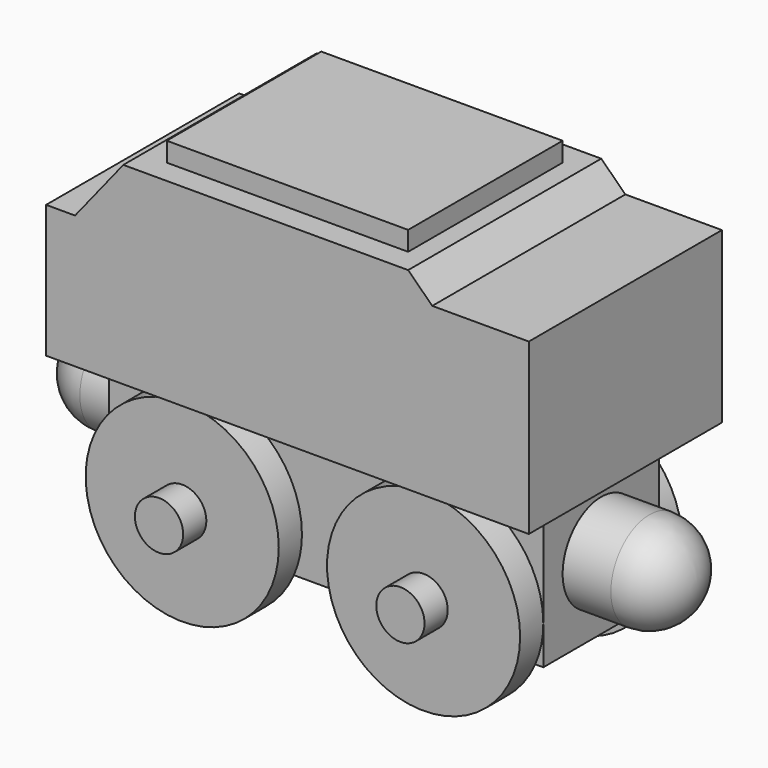
from build123d import *

# Parameters (mm, degrees)
F0_W      = 45
F0_H      = 15
F1_DEPTH  = 7.5
F2_W      = 50
F2_H      = 25
F3_DEPTH  = 20
F5_DEPTH  = 25
F7_DEPTH  = 25
F8_W      = 25
F8_H      = 20
F9_DEPTH  = 2
F11_W     = 5
F11_H     = 5
F13_W     = 5
F13_H     = 5
F15_R     = 10
F16_DEPTH = 3
F17_R     = 10
F18_DEPTH = 3
F19_R     = 2.5
F20_DEPTH = 3
F21_R     = 2.5
F22_DEPTH = 3


# Not quite as in the source:
# - a pattern or mirror of a feature is missing from the dataset's text; its kind, count and spacing are read off the source's solid


with BuildPart() as f1:
    # F0 (on Top) → F1 (new body, symmetric)
    with BuildSketch(Plane.XY):
        Rectangle(F0_W, F0_H)
    extrude(amount=F1_DEPTH, both=True)

    # F2 (on face) → F3 (join)
    with BuildSketch(Plane.XY.offset(7.5)):
        Rectangle(F2_W, F2_H)
    extrude(amount=F3_DEPTH)

    # F4 (on face) → F5 (cut, through all)
    with BuildSketch(Plane.XZ.offset(12.5)):
        Polygon((25, 27.5), (12.5, 27.5), (15, 25.0505102572), (25, 25.0505102572), align=None)
    extrude(amount=-F5_DEPTH, mode=Mode.SUBTRACT)

    # F6 (on face) → F7 (cut, through all)
    with BuildSketch(Plane.XZ.offset(12.5)):
        Polygon((-25, 27.5), (-25, 21.2550020016), (-22, 21.2550020016), (-17, 27.5), align=None)
    extrude(amount=-F7_DEPTH, mode=Mode.SUBTRACT)

    # F8 (on face) → F9 (join)
    with BuildSketch(Plane.XY.offset(27.5)):
        with Locations((-2, 0)):
            Rectangle(F8_W, F8_H)
    extrude(amount=F9_DEPTH)

    # F11 (on Front) → F12 (revolve)
    with BuildSketch(Plane.XZ):
        with Locations((25, -2.5)):
            Rectangle(F11_W, F11_H)
    revolve(axis=Axis((-8.4795374423, 0, 0), (-1, 0, 0)))

    # F13 (on Front) → F14 (revolve)
    with BuildSketch(Plane.XZ):
        with Locations((-25, -2.5)):
            Rectangle(F13_W, F13_H)
    revolve(axis=Axis((-8.4795374423, 0, 0), (-1, 0, 0)))

    # F15 (on face) → F16 (join)
    with BuildSketch(Plane.XZ.offset(7.5)):
        with Locations((-12.5, -3.5)):
            Circle(F15_R)
    f16 = extrude(amount=F16_DEPTH)

    # F16_copies: F16 across plane
    add(f16.mirror(Plane.ZX))

    # F17 (on face) → F18 (join)
    with BuildSketch(Plane.XZ.offset(7.5)):
        with Locations((12.5, -3.5)):
            Circle(F17_R)
    f18 = extrude(amount=F18_DEPTH)

    # F18_copies: F18 across plane
    add(f18.mirror(Plane.ZX))

    # F19 (on face) → F20 (join)
    with BuildSketch(Plane.XZ.offset(10.5)):
        with Locations((-12.5, -3.5)):
            Circle(F19_R)
    f20 = extrude(amount=F20_DEPTH)

    # F20_copies: F20 across plane
    add(f20.mirror(Plane.ZX))

    # F21 (on face) → F22 (join)
    with BuildSketch(Plane.XZ.offset(10.5)):
        with Locations((12.5, -3.5)):
            Circle(F21_R)
    f22 = extrude(amount=F22_DEPTH)

    # F22_copies: F22 across plane
    add(f22.mirror(Plane.ZX))

    # F23 (on Front) → F24 (revolve)
    with BuildSketch(Plane.XZ):
        with BuildLine():
            Line((-27.5, 0), (-27.5, 5))
            ThreePointArc((-27.5, 5), (-31.0355339059, 3.5355339059), (-32.5, 0))
            Line((-32.5, 0), (-27.5, 0))
        make_face()
    f24 = revolve(axis=Axis((-30, 0, 0), (1, 0, 0)))

    # F24_copies: F24 across plane
    add(f24.mirror(Plane(origin=(0, 0, 0), x_dir=(0, 0, 1), z_dir=(1, 0, 0))))


solid = f1.part
